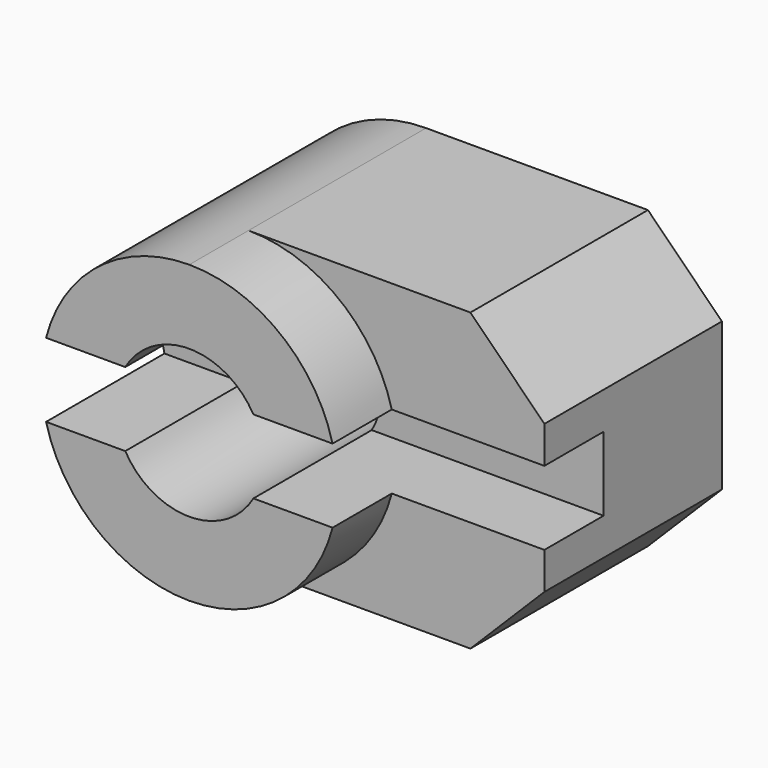
from build123d import *

# Parameters (mm, degrees)
F1_DEPTH = 15
F0_R     = 5
F2_DEPTH = 20
F4_DEPTH = 10


with BuildPart() as f1:
    # F0 (on Front) → F1 (new body)
    with BuildSketch(Plane.XZ):
        with BuildLine():
            ThreePointArc((0, 10), (7.0710678119, 7.0710678119), (10, 0))
            ThreePointArc((10, 0), (7.0710678119, -7.0710678119), (0, -10))
            Line((0, -10), (15, -10))
            Line((15, -10), (20, -5))
            Line((20, -5), (20, 5))
            Line((20, 5), (15, 10))
            Line((15, 10), (0, 10))
        make_face()
    extrude(amount=F1_DEPTH)

    # F0 (on Front) → F2 (join)
    with BuildSketch(Plane.XZ):
        with BuildLine():
            ThreePointArc((0, -10), (7.0710678119, -7.0710678119), (10, 0))
            ThreePointArc((10, 0), (7.0710678119, 7.0710678119), (0, 10))
            ThreePointArc((0, 10), (-10, 0), (0, -10))
        make_face()
        Circle(F0_R, mode=Mode.SUBTRACT)
    extrude(amount=F2_DEPTH)

    # F3 (on face) → F4 (cut)
    with BuildSketch(Plane.XZ.offset(20)):
        with BuildLine():
            Line((-4.3301270189, 2.5), (-9.6824583655, 2.5))
            ThreePointArc((-9.6824583655, 2.5), (-9.9202969627, 1.2600429248), (-10, 0))
            ThreePointArc((-10, 0), (-9.9202969627, -1.2600429248), (-9.6824583655, -2.5))
            Line((-9.6824583655, -2.5), (-4.3301270189, -2.5))
            ThreePointArc((-4.3301270189, -2.5), (-5, 0), (-4.3301270189, 2.5))
        make_face()
        with BuildLine():
            ThreePointArc((10, 0), (9.9202969627, 1.2600429248), (9.6824583655, 2.5))
            Line((9.6824583655, 2.5), (4.3301270189, 2.5))
            ThreePointArc((4.3301270189, 2.5), (4.8296291314, 1.2940952255), (5, 0))
            ThreePointArc((5, 0), (4.8296291314, -1.2940952255), (4.3301270189, -2.5))
            Line((4.3301270189, -2.5), (9.6824583655, -2.5))
            ThreePointArc((9.6824583655, -2.5), (9.9202969627, -1.2600429248), (10, 0))
        make_face()
        with BuildLine():
            Line((20, 2.5), (9.6824583655, 2.5))
            ThreePointArc((9.6824583655, 2.5), (9.9202969627, 1.2600429248), (10, 0))
            ThreePointArc((10, 0), (9.9202969627, -1.2600429248), (9.6824583655, -2.5))
            Line((9.6824583655, -2.5), (20, -2.5))
            Line((20, -2.5), (20, 0))
            Line((20, 0), (20, 2.5))
        make_face()
    extrude(amount=-F4_DEPTH, mode=Mode.SUBTRACT)


solid = f1.part
